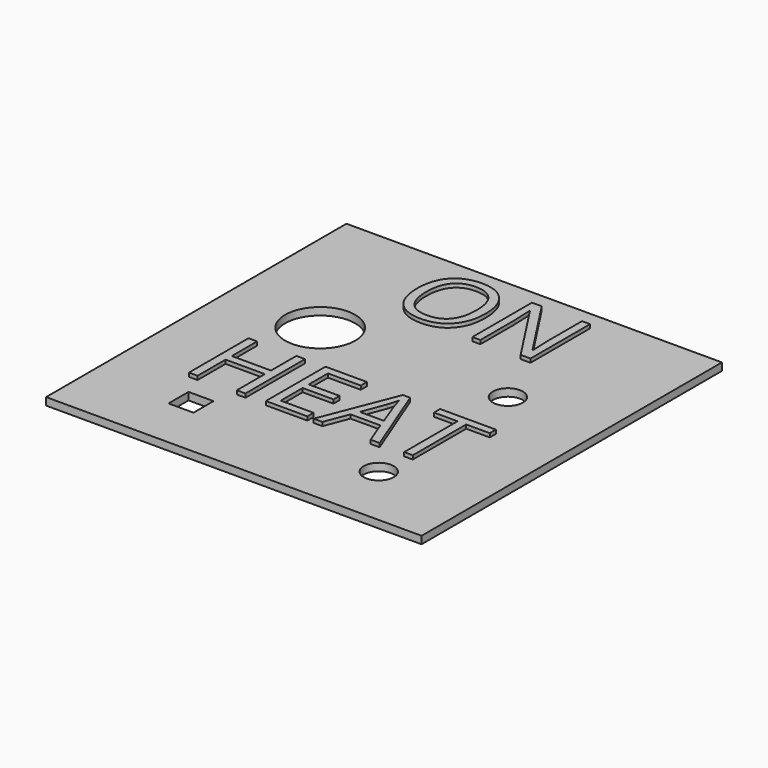
from build123d import *

# Parameters (mm, degrees)
F1_W         = 75
F1_H         = 75
F2_DEPTH     = 1.5
F3_TEXT_SIZE = 20.8333333333
F4_DEPTH     = 0.75
F5_R         = 7
F6_DEPTH     = 25
F7_R         = 7
F7_R_2       = 3
F8_DEPTH     = 25
F9_TEXT_SIZE = 20.8333333333
F10_DEPTH    = 0.75
F11_R        = 5
F11_R_2      = 7
F11_R_3      = 3
F12_DEPTH    = 25
F13_R        = 5
F14_DEPTH    = 1.5
F15_W        = 5
F15_H        = 5
F16_DEPTH    = 25


# Not quite as in the source:
# - Text() gives the source's letters only with a copy of the font that has no kerning and outlines rounded to 1/6400 em; it was checked with that copy


with BuildPart() as f2:
    # F1 (on Top) → F2 (new body)
    with BuildSketch(Plane.XY):
        with Locations((-14.0325602144, 2.8565365667)):
            Rectangle(F1_W, F1_H)
    extrude(amount=F2_DEPTH)

    # F3 (on face) → F4 (join)
    with BuildSketch(Plane.XY.offset(1.5)):
        with Locations((-29.6510497977, 21.6065365667)):
            Text('ON', F3_TEXT_SIZE, font='Open Sans', text_align=(TextAlign.LEFT, TextAlign.BOTTOM))
    extrude(amount=F4_DEPTH)

    # F5 (on face) → F6 (cut)
    with BuildSketch(Plane.XY.offset(1.5)):
        with Locations((-32.7825602144, 10.3565365667)):
            Circle(F5_R)
    extrude(amount=-F6_DEPTH, mode=Mode.SUBTRACT)

    # F7 (on face) → F8 (cut)
    with BuildSketch(Plane.XY.offset(1.5)):
        with Locations((-32.7825602144, 10.3565365667)):
            Circle(F7_R)
        with Locations((4.7174397856, 10.3565365667)):
            Circle(F7_R_2)
    extrude(amount=-F8_DEPTH, mode=Mode.SUBTRACT)

    # F9 (on face) → F10 (join)
    with BuildSketch(Plane.XY.offset(1.5)):
        with Locations((-40.4436930269, -15.3934634333)):
            Text('HEAT', F9_TEXT_SIZE, font='Open Sans', text_align=(TextAlign.LEFT, TextAlign.BOTTOM))
    extrude(amount=F10_DEPTH)

    # F11 (on face) → F12 (cut)
    with BuildSketch(Plane.XY.offset(1.5)):
        with Locations((-32.7825602144, -21.8934634333)):
            Circle(F11_R)
        with Locations((-32.7825602144, 10.3565365667)):
            Circle(F11_R_2)
        with Locations((4.7174397856, -21.8934634333)):
            Circle(F11_R_3)
        with Locations((4.7174397856, 10.3565365667)):
            Circle(F11_R_3)
    extrude(amount=-F12_DEPTH, mode=Mode.SUBTRACT)

    # F13 (on face) → F14 (join, through all)
    with BuildSketch(Plane.XY.offset(1.5)):
        with Locations((-32.7825602144, -21.8934634333)):
            Circle(F13_R)
    extrude(amount=-F14_DEPTH)

    # F15 (on face) → F16 (cut)
    with BuildSketch(Plane.XY.offset(1.5)):
        with Locations((-32.7825602144, -21.8934634333)):
            Rectangle(F15_W, F15_H)
    extrude(amount=-F16_DEPTH, mode=Mode.SUBTRACT)


solid = f2.part
